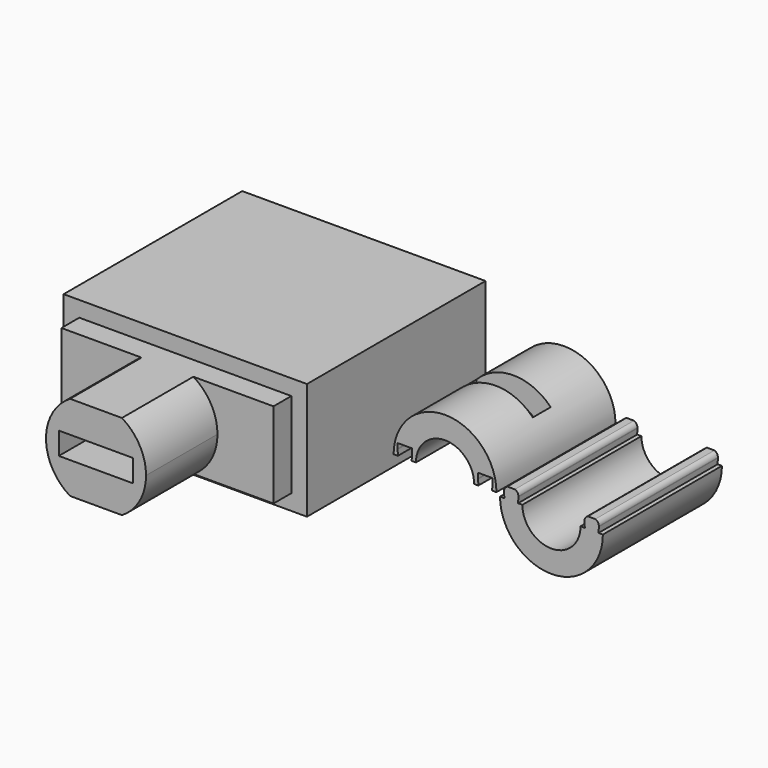
from build123d import *

# Parameters (mm, degrees)
F0_W     = 16.35
F0_H     = 7.85
F1_DEPTH = 7.5
F0_W_2   = 5
F0_H_2   = 1.5
F2_DEPTH = 9
F3_DEPTH = 15
F4_DEPTH = 5
F5_W     = 5
F5_H     = 1.5
F6_DEPTH = 9.752


with BuildPart() as f1:
    # F0 (on Front) → F1 (new body, symmetric)
    with BuildSketch(Plane.XZ):
        Rectangle(F0_W, F0_H)
        with BuildLine():
            Line((1.7415829263, 2.875), (7.125, 2.875))
            Line((7.125, 2.875), (7.125, -2.875))
            Line((7.125, -2.875), (1.7415829263, -2.875))
            ThreePointArc((1.7415829263, -2.875), (0, -3.3613592622), (-1.7415829263, -2.875))
            Line((-1.7415829263, -2.875), (-7.125, -2.875))
            Line((-7.125, -2.875), (-7.125, 2.875))
            Line((-7.125, 2.875), (-1.7415829263, 2.875))
            ThreePointArc((-1.7415829263, 2.875), (0, 3.3613592622), (1.7415829263, 2.875))
        make_face(mode=Mode.SUBTRACT)
        with BuildLine():
            ThreePointArc((-1.7415829263, -2.875), (0, -3.3613592622), (1.7415829263, -2.875))
            Line((1.7415829263, -2.875), (-1.7415829263, -2.875))
        make_face()
        with BuildLine():
            Line((-1.7415829263, 2.875), (1.7415829263, 2.875))
            ThreePointArc((1.7415829263, 2.875), (0, 3.3613592622), (-1.7415829263, 2.875))
        make_face()
    extrude(amount=F1_DEPTH, both=True)

    # F0 (on Front) → F2 (join)
    with BuildSketch(Plane.XZ):
        with BuildLine():
            Line((7.125, -2.875), (7.125, 2.875))
            Line((7.125, 2.875), (1.7415829263, 2.875))
            ThreePointArc((1.7415829263, 2.875), (2.928551006, 1.6499469975), (3.3613592622, 0))
            ThreePointArc((3.3613592622, 0), (2.928551006, -1.6499469975), (1.7415829263, -2.875))
            Line((1.7415829263, -2.875), (7.125, -2.875))
        make_face()
        with BuildLine():
            ThreePointArc((3.3613592622, 0), (2.928551006, 1.6499469975), (1.7415829263, 2.875))
            Line((1.7415829263, 2.875), (-1.7415829263, 2.875))
            ThreePointArc((-1.7415829263, 2.875), (-3.3613592622, 0), (-1.7415829263, -2.875))
            Line((-1.7415829263, -2.875), (1.7415829263, -2.875))
            ThreePointArc((1.7415829263, -2.875), (2.928551006, -1.6499469975), (3.3613592622, 0))
        make_face()
        Rectangle(F0_W_2, F0_H_2, mode=Mode.SUBTRACT)
        with BuildLine():
            ThreePointArc((-1.7415829263, -2.875), (-3.3613592622, 0), (-1.7415829263, 2.875))
            Line((-1.7415829263, 2.875), (-7.125, 2.875))
            Line((-7.125, 2.875), (-7.125, -2.875))
            Line((-7.125, -2.875), (-1.7415829263, -2.875))
        make_face()
        Rectangle(F0_W_2, F0_H_2)
    extrude(amount=F2_DEPTH)

    # F0 (on Front) → F3 (join)
    with BuildSketch(Plane.XZ):
        with BuildLine():
            ThreePointArc((3.3613592622, 0), (2.928551006, 1.6499469975), (1.7415829263, 2.875))
            Line((1.7415829263, 2.875), (-1.7415829263, 2.875))
            ThreePointArc((-1.7415829263, 2.875), (-3.3613592622, 0), (-1.7415829263, -2.875))
            Line((-1.7415829263, -2.875), (1.7415829263, -2.875))
            ThreePointArc((1.7415829263, -2.875), (2.928551006, -1.6499469975), (3.3613592622, 0))
        make_face()
        Rectangle(F0_W_2, F0_H_2, mode=Mode.SUBTRACT)
    extrude(amount=F3_DEPTH)


with BuildPart() as f4:
    # F0 (on Front) → F4 (new body, symmetric)
    with BuildSketch(Plane.XZ):
        with BuildLine():
            ThreePointArc((13.4986763668, 0), (15.4536763668, 1.955), (17.4086763668, 0))
            Line((17.4086763668, 0), (17.6948876991, 0))
            Line((17.6948876991, 0), (17.676782033, 0.375))
            ThreePointArc((17.676782033, 0.375), (17.6753254742, 0.3943374538), (17.6749123074, 0.4137252844))
            Line((17.6749123074, 0.4137252844), (17.6586763668, 0.75))
            Line((17.6586763668, 0.75), (18.6586763668, 0.75))
            Line((18.6586763668, 0.75), (18.6405108834, 0.4100266558))
            ThreePointArc((18.6405108834, 0.4100266558), (18.6400019662, 0.3924905201), (18.6386393362, 0.375))
            Line((18.6386393362, 0.375), (18.6186023057, 0))
            Line((18.6186023057, 0), (18.9086763668, 0))
            ThreePointArc((18.9086763668, 0), (15.4536763668, 3.455), (11.9986763668, 0))
            Line((11.9986763668, 0), (12.288750428, 0))
            Line((12.288750428, 0), (12.2687133974, 0.375))
            ThreePointArc((12.2687133974, 0.375), (12.2673507674, 0.3924905201), (12.2668418503, 0.4100266558))
            Line((12.2668418503, 0.4100266558), (12.2486763668, 0.75))
            Line((12.2486763668, 0.75), (13.2486763668, 0.75))
            Line((13.2486763668, 0.75), (13.2324404262, 0.4137252844))
            ThreePointArc((13.2324404262, 0.4137252844), (13.2320272594, 0.3943374538), (13.2305707006, 0.375))
            Line((13.2305707006, 0.375), (13.2124650345, 0))
            Line((13.2124650345, 0), (13.4986763668, 0))
        make_face()
    extrude(amount=F4_DEPTH, both=True)

    # F5 (on Top) → F6 (cut)
    with BuildSketch(Plane.XY):
        with Locations((15.4536763668, 0)):
            Rectangle(F5_W, F5_H)
    extrude(amount=F6_DEPTH, mode=Mode.SUBTRACT)


with BuildPart() as f4b:
    # F0 (on Front) → F4, piece 2 (new body, symmetric)
    with BuildSketch(Plane.XZ):
        with BuildLine():
            Line((19.440587234, -0.1789705101), (19.1505131729, -0.1789705101))
            ThreePointArc((19.1505131729, -0.1789705101), (19.3207003873, -1.2499653577), (19.8144957857, -2.2154495658))
            ThreePointArc((19.8144957857, -2.2154495658), (20.0606948092, -2.5158326147), (20.3390517964, -2.7866855691))
            ThreePointArc((20.3390517964, -2.7866855691), (22.6055131729, -3.6339705101), (24.8719745493, -2.7866855691))
            ThreePointArc((24.8719745493, -2.7866855691), (25.7493682153, -1.6118698339), (26.0605131729, -0.1789705101))
            Line((26.0605131729, -0.1789705101), (25.7704391117, -0.1789705101))
            Line((25.7704391117, -0.1789705101), (25.7904761423, 0.1960294899))
            Line((25.7904761423, 0.1960294899), (25.7923476894, 0.2310561457))
            ThreePointArc((25.7923476894, 0.2310561457), (25.7277150085, 0.4385446809), (25.5554458847, 0.5710294899))
            Line((25.5554458847, 0.5710294899), (25.0636490966, 0.5710294899))
            ThreePointArc((25.0636490966, 0.5710294899), (24.8924411463, 0.4400592427), (24.8267491135, 0.2347547743))
            Line((24.8267491135, 0.2347547743), (24.828618839, 0.1960294899))
            Line((24.828618839, 0.1960294899), (24.8467245052, -0.1789705101))
            Line((24.8467245052, -0.1789705101), (24.5605131729, -0.1789705101))
            ThreePointArc((24.5605131729, -0.1789705101), (24.4721322835, -0.7601401032), (24.2149805939, -1.2887631126))
            ThreePointArc((24.2149805939, -1.2887631126), (22.3860935077, -2.1216181906), (20.789052355, -0.9018087335))
            ThreePointArc((20.789052355, -0.9018087335), (20.6854603222, -0.5469678614), (20.6505131729, -0.1789705101))
            Line((20.6505131729, -0.1789705101), (20.3643018405, -0.1789705101))
            Line((20.3643018405, -0.1789705101), (20.3824075067, 0.1960294899))
            Line((20.3824075067, 0.1960294899), (20.3842772322, 0.2347547743))
            ThreePointArc((20.3842772322, 0.2347547743), (20.3185851995, 0.4400592427), (20.1473772491, 0.5710294899))
            Line((20.1473772491, 0.5710294899), (19.655580461, 0.5710294899))
            ThreePointArc((19.655580461, 0.5710294899), (19.4833113372, 0.4385446809), (19.4186786563, 0.2310561457))
            Line((19.4186786563, 0.2310561457), (19.4205502034, 0.1960294899))
            Line((19.4205502034, 0.1960294899), (19.440587234, -0.1789705101))
        make_face()
    extrude(amount=F4_DEPTH, both=True)


solid = Compound([f1.part, f4.part, f4b.part])
